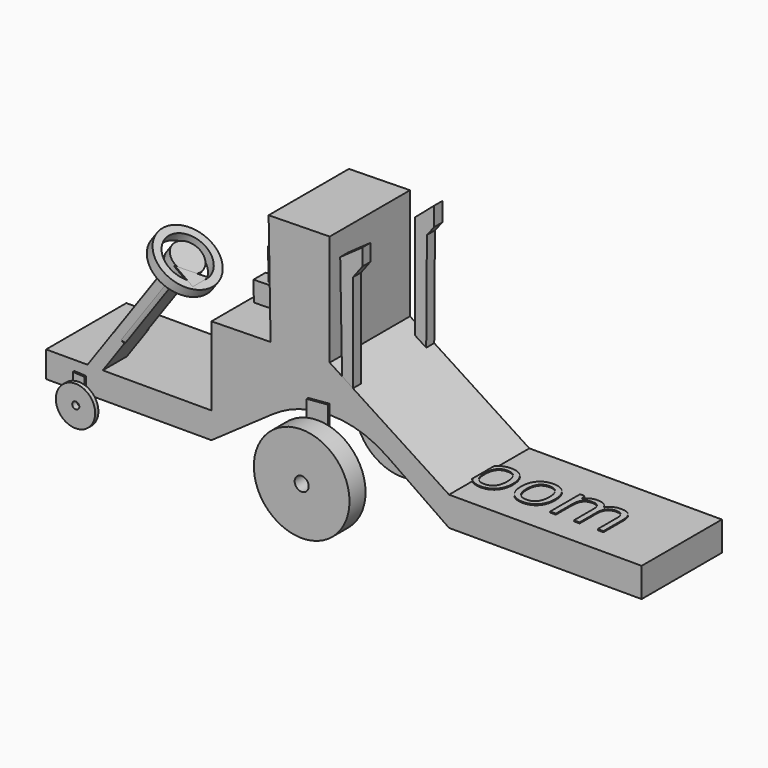
from build123d import *

# Parameters (mm, degrees)
F1_DEPTH      = 25.4
F3_DEPTH      = 0.508
F5_DEPTH      = 0.508
F6_R          = 12.1072853721
F7_DEPTH      = 5.08
F8_R          = 11.9218090621
F9_DEPTH      = 5.08
F11_DEPTH     = 7.62
F12_R         = 7.7678656061
F13_DEPTH     = 2.54
F14_R         = 5.7817793367
F14_R_2       = 3.9431965494
F15_DEPTH     = 25.4
F17_DEPTH     = 0.254
F18_TEXT_SIZE = 17.6423184005
F19_DEPTH     = 0.254
F22_DEPTH     = 2.54
F23_DEPTH     = 2.54
F25_DEPTH     = 5.08
F26_R         = 1.2709260418
F27_DEPTH     = 7.62
F28_R         = 1.7723311016
F29_DEPTH     = 36.577
F31_W         = 3.4198537469
F31_H         = 9.0700322762
F32_DEPTH     = 0.508
F33_DEPTH     = 0.508
F34_R         = 4.9790397539
F35_DEPTH     = 1.016
F36_R         = 5.0319069594
F37_DEPTH     = 1.016
F38_R         = 0.8959562409
F39_DEPTH     = 32.513


# Not quite as in the source:
# - Text() gives the source's letters only with a copy of the font that has no kerning and outlines rounded to 1/6400 em; it was checked with that copy


with BuildPart() as f1:
    # F0 (on Front) → F1 (new body)
    with BuildSketch(Plane.XZ):
        with BuildLine():
            Line((-71.7970505357, 23.3114119619), (-71.7970505357, 16.6880693287))
            Line((-71.7970505357, 16.6880693287), (-29.9375168979, 16.6880693287))
            Line((-29.9375168979, 16.6880693287), (-14.489652701, 27.4879027482))
            ThreePointArc((-14.489652701, 27.4879027482), (0.0114580274, 32.0707061735), (14.5313772066, 27.5478479376))
            Line((14.5313772066, 27.5478479376), (30.2024520934, 16.6880693287))
            Line((30.2024520934, 16.6880693287), (78.9502710104, 16.6880693287))
            Line((78.9502710104, 16.6880693287), (78.9502710104, 24.106213823))
            Line((78.9502710104, 24.106213823), (30.2024520934, 24.106213823))
            Line((30.2024520934, 24.106213823), (0, 43.7113121152))
            Line((0, 43.7113121152), (-29.9375168979, 23.3114119619))
            Line((-29.9375168979, 23.3114119619), (-71.7970505357, 23.3114119619))
        make_face()
        Polygon((-29.9375168979, 43.1814491749), (-29.9375168979, 23.3114119619), (0, 43.7113121152), (-14.968758449, 43.446380645), align=None)
        Polygon((-14.968758449, 43.446380645), (0, 43.7113121152), (0, 71.8013236791), (-15.4657667752, 71.527595678), align=None)
    extrude(amount=F1_DEPTH)

    # F2 (on face) → F3 (join)
    with BuildSketch(Plane.XZ.offset(25.4)):
        Polygon((0, 34.5462113619), (-5.4421040953, 34.073620886), (-5.4421040953, 31.4668015587), (-5.4421040953, 14.3822990358), (0, 14.3822990358), align=None)
    extrude(amount=F3_DEPTH)

    # F4 (on face) → F5 (join)
    with BuildSketch(Plane(origin=(0, 0, 0), x_dir=(-1, 0, 0), z_dir=(0, 1, 0))):
        Polygon((5.4241362959, 33.7585583329), (0, 33.9160896838), (0, 14.5398294553), (5.4241362959, 14.5398294553), align=None)
    extrude(amount=F5_DEPTH)

    # F6 (on face) → F7 (join)
    with BuildSketch(Plane.XZ.offset(25.908)):
        with Locations((-2.6304533239, 18.1199219078)):
            Circle(F6_R)
    extrude(amount=F7_DEPTH)

    # F8 (on face) → F9 (join)
    with BuildSketch(Plane(origin=(0, 0.508, 0), x_dir=(-1, 0, 0), z_dir=(0, 1, 0))):
        with Locations((2.4082383607, 18.8280101866)):
            Circle(F8_R)
    extrude(amount=F9_DEPTH)

    # F10 (on face) → F11 (join)
    with BuildSketch(Plane.XZ.offset(25.4)):
        Polygon((-41.4261519909, 51.5343733132), (-61.3062530756, 23.3114119619), (-57.4475711594, 23.3114119619), (-38.8471152109, 49.7177137767), align=None)
    extrude(amount=-F11_DEPTH)

    # F12 (on face) → F13 (join)
    with BuildSketch(Plane(origin=(10.5242250367, 0, 14.9408091637), x_dir=(0.8175405032, 0, -0.5758711016), z_dir=(0.5758711016, 0, 0.8175405032))):
        with Locations((-62.3752214015, -21.59)):
            Circle(F12_R)
    extrude(amount=F13_DEPTH)

    # F14 (on face) → F15 (cut)
    with BuildSketch(Plane(origin=(11.9869376347, 0, 17.0173620418), x_dir=(0.8175405032, 0, -0.5758711016), z_dir=(0.5758711016, 0, 0.8175405032))):
        with Locations((-62.3752214015, -21.59)):
            Circle(F14_R)
        with Locations((-62.3752214015, -21.59)):
            Circle(F14_R_2, mode=Mode.SUBTRACT)
    extrude(amount=-F15_DEPTH, mode=Mode.SUBTRACT)

    # F18 (on face) → F19 (join)
    with BuildSketch(Plane.XY.offset(24.106213823)):
        with Locations((10.0747346878, -18.8982887194)):
            Text('Vroom', F18_TEXT_SIZE, font='Open Sans', text_align=(TextAlign.LEFT, TextAlign.BOTTOM))
    extrude(amount=F19_DEPTH)

    # F21 (on face) → F22 (join)
    with BuildSketch(Plane(origin=(0, 0, 0), x_dir=(-1, 0, 0), z_dir=(0, 1, 0))):
        Polygon((-6.3079516403, 64.9060159922), (-6.1318677613, 39.7309773462), (-3.2345788028, 41.6116734777), (-3.2345788028, 67.8202882409), (-8.1624891609, 72.0592290163), (-8.1624891609, 67.29041785), align=None)
    extrude(amount=-F22_DEPTH)

    # F20 (on face) → F23 (join)
    with BuildSketch(Plane.XZ.offset(25.4)):
        Polygon((2.6518103364, 68.0937521038), (3.1191899305, 41.686575018), (5.8790105395, 39.8951127175), (5.8790105395, 64.6410807967), (8.2634137943, 67.8202882409), (8.2634137943, 72.0592290163), align=None)
    extrude(amount=-F23_DEPTH)

    # F24 (on face) → F25 (join)
    with BuildSketch(Plane(origin=(-0.7734025322, 0, 43.697623694), x_dir=(0.9998434102, 0, 0.0176961894), z_dir=(-0.0176961894, 0, 0.9998434102))):
        Polygon((-14.1975791132, -13.9321908355), (-14.1975791132, -10.0887026638), (-22.5263908505, -10.0887026638), (-27.6087280363, -10.0887026638), (-27.6087280363, -13.9321908355), (-22.5263908505, -13.9321908355), align=None)
    extrude(amount=F25_DEPTH)

    # F26 (on face) → F27 (join)
    with BuildSketch(Plane(origin=(-0.8632991743, 0, 48.7768282177), x_dir=(0.9998434102, 0, 0.0176961894), z_dir=(-0.0176961894, 0, 0.9998434102))):
        with Locations((-23.8041765988, -11.8869105354)):
            Circle(F26_R)
    extrude(amount=F27_DEPTH)

    # F28 (on face) → F29 (cut, through all)
    with BuildSketch(Plane.XZ.offset(30.988)):
        with Locations((-2.6304533239, 18.1199219078)):
            Circle(F28_R)
    extrude(amount=-F29_DEPTH, mode=Mode.SUBTRACT)

    # F31 (on face) → F32 (join)
    with BuildSketch(Plane(origin=(0, 0, 0), x_dir=(-1, 0, 0), z_dir=(0, 1, 0))):
        with Locations((63.259806484, 16.4483594708)):
            Rectangle(F31_W, F31_H)
    extrude(amount=F32_DEPTH)

    # F30 (on face) → F33 (join)
    with BuildSketch(Plane.XZ.offset(25.4)):
        Polygon((-61.6394802928, 20.6859968603), (-64.6132603288, 20.8346862346), (-64.6132603288, 11.6159655154), (-61.6394802928, 11.6159655154), align=None)
    extrude(amount=F33_DEPTH)

    # F34 (on face) → F35 (join)
    with BuildSketch(Plane.XZ.offset(25.908)):
        with Locations((-63.131660223, 14.1321774572)):
            Circle(F34_R)
    extrude(amount=F35_DEPTH)

    # F36 (on face) → F37 (join)
    with BuildSketch(Plane(origin=(0, 0.508, 0), x_dir=(-1, 0, 0), z_dir=(0, 1, 0))):
        with Locations((63.06399405, 14.2767829821)):
            Circle(F36_R)
    extrude(amount=F37_DEPTH)

    # F38 (on face) → F39 (cut, through all)
    with BuildSketch(Plane(origin=(0, 1.524, 0), x_dir=(-1, 0, 0), z_dir=(0, 1, 0))):
        with Locations((63.06399405, 14.2767829821)):
            Circle(F38_R)
    extrude(amount=-F39_DEPTH, mode=Mode.SUBTRACT)


with BuildPart() as f17:
    # F16 (on face) → F17 (new body)
    with BuildSketch(Plane(origin=(11.9869376347, 0, 17.0173620418), x_dir=(0.8175405032, 0, -0.5758711016), z_dir=(0.5758711016, 0, 0.8175405032))):
        Polygon((-60.6327201668, -24.458463907), (-62.2241513694, -25.8239789062), (-56.6508824471, -25.8239789062), (-56.6508824471, -20.7770326981), align=None)
    extrude(amount=-F17_DEPTH)


solid = Compound([f1.part, f17.part])
